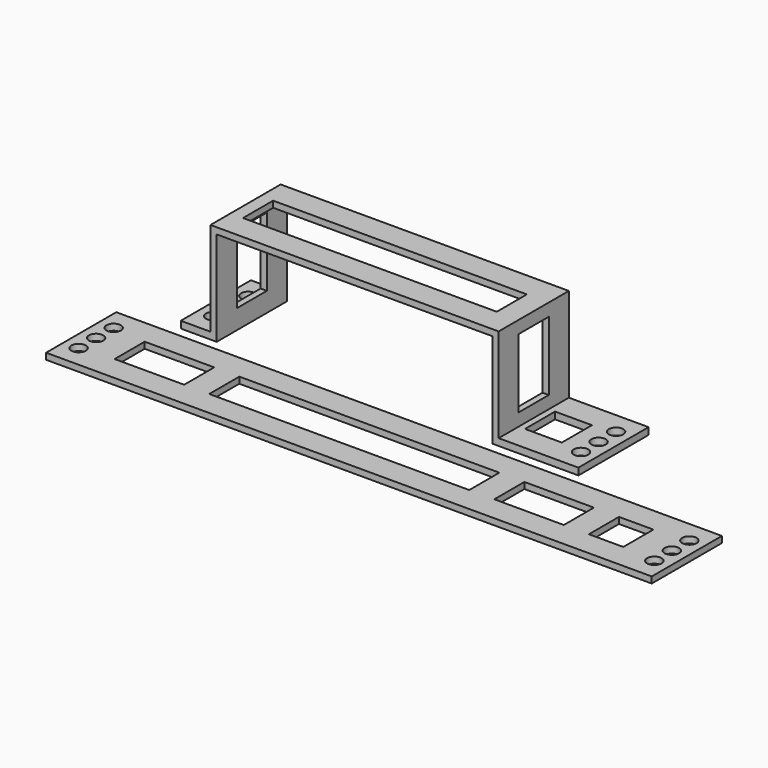
from build123d import *

# Parameters (mm, degrees)
F0_W      = 105.41
F0_H      = 10.16
F0_W_2    = 26.6446
F0_H_2    = 15.24
F0_R      = 2.921
F1_DEPTH  = 40.894
F2_W      = 12.0396
F2_H      = 35.56
F2_R      = 2.921
F2_W_2    = 32.3342
F3_DEPTH  = 38.1
F4_W      = 105.41
F4_H      = 10.16
F4_W_2    = 1.27
F4_H_2    = 35.56
F5_DEPTH  = 38.354
F6_W      = 15.24
F6_H      = 27.94
F7_DEPTH  = 149.1752
F8_W      = 14.9580658293
F8_H      = 15.24
F9_DEPTH  = 5.08
F10_W     = 14.5796
F10_H     = 35.56
F10_R     = 2.921
F10_W_2   = 38.354
F10_W_3   = 28.194
F10_H_2   = 15.24
F10_W_4   = 115.57
F10_W_5   = 105.41
F10_W_6   = 24.1046
F10_W_7   = 13.9446
F11_DEPTH = 2.54
F12_W     = 15.24
F12_H     = 2.54
F13_DEPTH = 2.54


with BuildPart() as f1:
    # F0 (on Top) → F1 (new body)
    with BuildSketch(Plane.XY):
        with Locations((-13.3223, 12.7)):
            Rectangle(F0_W, F0_H)
        with BuildLine():
            Line((-66.0273, 7.62), (-66.0273, 17.78))
            Line((-66.0273, 17.78), (-74.549, 17.78))
            Line((-74.549, 17.78), (-74.549, 11.811))
            ThreePointArc((-74.549, 11.811), (-72.4835410922, 10.9554589078), (-71.628, 8.89))
            ThreePointArc((-71.628, 8.89), (-72.4835410922, 6.8245410922), (-74.549, 5.969))
            Line((-74.549, 5.969), (-74.549, 2.921))
            ThreePointArc((-74.549, 2.921), (-72.4835410922, 2.0654589078), (-71.628, 0))
            ThreePointArc((-71.628, 0), (-72.4835410922, -2.0654589078), (-74.549, -2.921))
            Line((-74.549, -2.921), (-74.549, -5.969))
            ThreePointArc((-74.549, -5.969), (-72.4835410922, -6.8245410922), (-71.628, -8.89))
            ThreePointArc((-71.628, -8.89), (-72.4835410922, -10.9554589078), (-74.549, -11.811))
            Line((-74.549, -11.811), (-74.549, -17.78))
            Line((-74.549, -17.78), (-66.0273, -17.78))
            Line((-66.0273, -17.78), (-66.0273, -7.62))
            Line((-66.0273, -7.62), (-66.0273, 7.62))
        make_face()
        with Locations((-13.3223, -12.7)):
            Rectangle(F0_W, F0_H)
        with Locations((52.705, -12.7)):
            Rectangle(F0_W_2, F0_H)
        with Locations((52.705, 12.7)):
            Rectangle(F0_W_2, F0_H)
        with Locations((52.705, 0)):
            Rectangle(F0_W_2, F0_H_2)
        Polygon((80.6069, -17.78), (80.6069, 17.78), (66.0273, 17.78), (66.0273, 7.62), (66.0273, -7.62), (66.0273, -17.78), align=None)
        with Locations((74.549, -8.89)):
            Circle(F0_R, mode=Mode.SUBTRACT)
        with Locations((74.549, 0)):
            Circle(F0_R, mode=Mode.SUBTRACT)
        with Locations((74.549, 8.89)):
            Circle(F0_R, mode=Mode.SUBTRACT)
        with BuildLine():
            Line((-74.549, 11.811), (-74.549, 17.78))
            Line((-74.549, 17.78), (-80.6069, 17.78))
            Line((-80.6069, 17.78), (-80.6069, 0))
            Line((-80.6069, 0), (-80.6069, -8.89))
            Line((-80.6069, -8.89), (-80.6069, -17.78))
            Line((-80.6069, -17.78), (-74.549, -17.78))
            Line((-74.549, -17.78), (-74.549, -11.811))
            ThreePointArc((-74.549, -11.811), (-77.47, -8.89), (-74.549, -5.969))
            Line((-74.549, -5.969), (-74.549, -2.921))
            ThreePointArc((-74.549, -2.921), (-77.47, 0), (-74.549, 2.921))
            Line((-74.549, 2.921), (-74.549, 5.969))
            ThreePointArc((-74.549, 5.969), (-77.47, 8.89), (-74.549, 11.811))
        make_face()
    extrude(amount=F1_DEPTH)

    # F2 (on face) → F3 (cut)
    with BuildSketch(Plane.XY.offset(40.894)):
        with Locations((-74.5871, 0)):
            Rectangle(F2_W, F2_H)
        with Locations((-74.549, -8.89)):
            Circle(F2_R, mode=Mode.SUBTRACT)
        with Locations((-74.549, 0)):
            Circle(F2_R, mode=Mode.SUBTRACT)
        with Locations((-74.549, 8.89)):
            Circle(F2_R, mode=Mode.SUBTRACT)
        with Locations((64.4398, 0)):
            Rectangle(F2_W_2, F2_H)
        with Locations((74.549, -8.89)):
            Circle(F2_R, mode=Mode.SUBTRACT)
        with Locations((74.549, 0)):
            Circle(F2_R, mode=Mode.SUBTRACT)
        with Locations((74.549, 8.89)):
            Circle(F2_R, mode=Mode.SUBTRACT)
    extrude(amount=-F3_DEPTH, mode=Mode.SUBTRACT)

    # F4 (on face) → F5 (cut)
    with BuildSketch(Plane(origin=(0, 0, 0), x_dir=(1, 0, 0), z_dir=(0, 0, -1))):
        with Locations((-13.3223, 12.7)):
            Rectangle(F4_W, F4_H)
        with Locations((-13.3223, -12.7)):
            Rectangle(F4_W, F4_H)
        Polygon((39.3827, 17.78), (39.3827, 7.62), (39.3827, -7.62), (39.3827, -17.78), (44.4627, -17.78), (44.4627, 17.78), align=None)
        with Locations((45.0977, 0)):
            Rectangle(F4_W_2, F4_H_2)
    extrude(amount=-F5_DEPTH, mode=Mode.SUBTRACT)

    # F6 (on face) → F7 (cut, through all)
    with BuildSketch(Plane(origin=(-68.5673, 0, 0), x_dir=(0, -1, 0), z_dir=(-1, 0, 0))):
        with Locations((0, 21.844)):
            Rectangle(F6_W, F6_H)
    extrude(amount=-F7_DEPTH, mode=Mode.SUBTRACT)

    # F8 (on face) → F9 (cut)
    with BuildSketch(Plane.XY.offset(2.794)):
        with Locations((58.2917329146, 0)):
            Rectangle(F8_W, F8_H)
    extrude(amount=-F9_DEPTH, mode=Mode.SUBTRACT)

    # F12 (on face) → F13 (join)
    with BuildSketch(Plane.YZ.offset(-66.0273)):
        with Locations((0, 39.624)):
            Rectangle(F12_W, F12_H)
    extrude(amount=F13_DEPTH)


with BuildPart() as f11:
    # F10 (on Top) → F11 (new body)
    with BuildSketch(Plane.XY):
        with Locations((-93.2281401838, -43.3592097834)):
            Rectangle(F10_W, F10_H)
        with Locations((-94.4473401838, -52.2492097834)):
            Circle(F10_R, mode=Mode.SUBTRACT)
        with Locations((-94.4473401838, -43.3592097834)):
            Circle(F10_R, mode=Mode.SUBTRACT)
        with Locations((-94.4473401838, -34.4692097834)):
            Circle(F10_R, mode=Mode.SUBTRACT)
        with Locations((-66.7613401838, -43.3592097834)):
            Rectangle(F10_W_2, F10_H)
        with Locations((-66.7613401838, -43.3592097834)):
            Rectangle(F10_W_3, F10_H_2, mode=Mode.SUBTRACT)
        with Locations((10.2006598162, -43.3592097834)):
            Rectangle(F10_W_4, F10_H)
        with Locations((10.2006598162, -43.3592097834)):
            Rectangle(F10_W_5, F10_H_2, mode=Mode.SUBTRACT)
        with Locations((87.1626598162, -43.3592097834)):
            Rectangle(F10_W_2, F10_H)
        with Locations((87.1626598162, -43.3592097834)):
            Rectangle(F10_W_3, F10_H_2, mode=Mode.SUBTRACT)
        with Locations((118.3919598162, -43.3592097834)):
            Rectangle(F10_W_6, F10_H)
        with Locations((118.3919598162, -43.3592097834)):
            Rectangle(F10_W_7, F10_H_2, mode=Mode.SUBTRACT)
        with Locations((137.7340598162, -43.3592097834)):
            Rectangle(F10_W, F10_H)
        with Locations((138.9532598162, -52.2492097834)):
            Circle(F10_R, mode=Mode.SUBTRACT)
        with Locations((138.9532598162, -43.3592097834)):
            Circle(F10_R, mode=Mode.SUBTRACT)
        with Locations((138.9532598162, -34.4692097834)):
            Circle(F10_R, mode=Mode.SUBTRACT)
    extrude(amount=F11_DEPTH)


solid = Compound([f1.part, f11.part])
